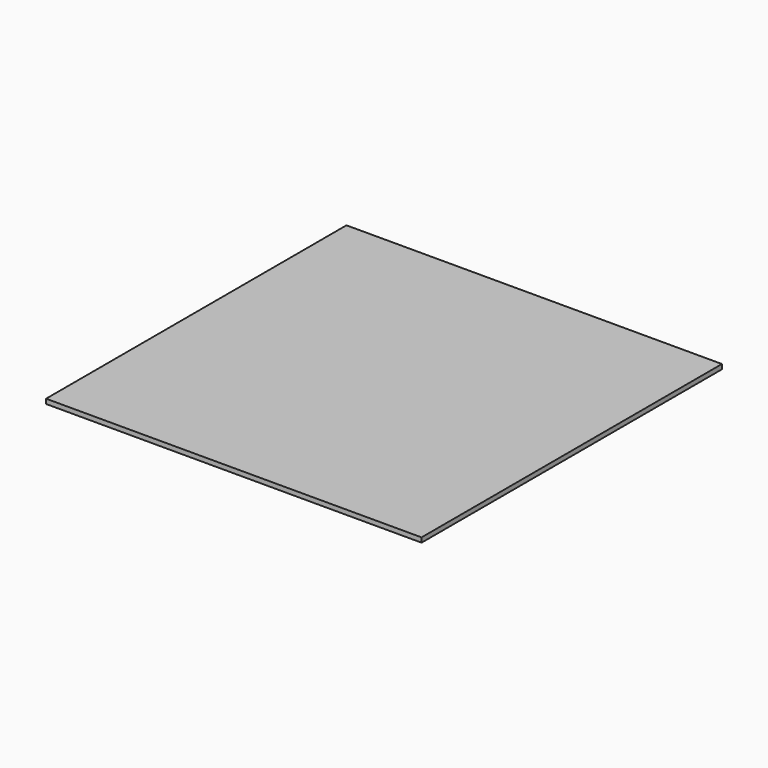
from build123d import *

# Parameters (mm, degrees)
F0_W     = 508
F0_H     = 508
F1_DEPTH = 6.35


# Not quite as in the source:
# - the program builds the solid bodies; features that only make, move or delete a surface that nothing else refers to are left out


with BuildPart() as f1:
    # F0 (on Top) → F1 (new body)
    with BuildSketch(Plane.XY):
        with Locations((-18.8210361949, 5.0480663776)):
            Rectangle(F0_W, F0_H)
    extrude(amount=F1_DEPTH)


solid = f1.part
